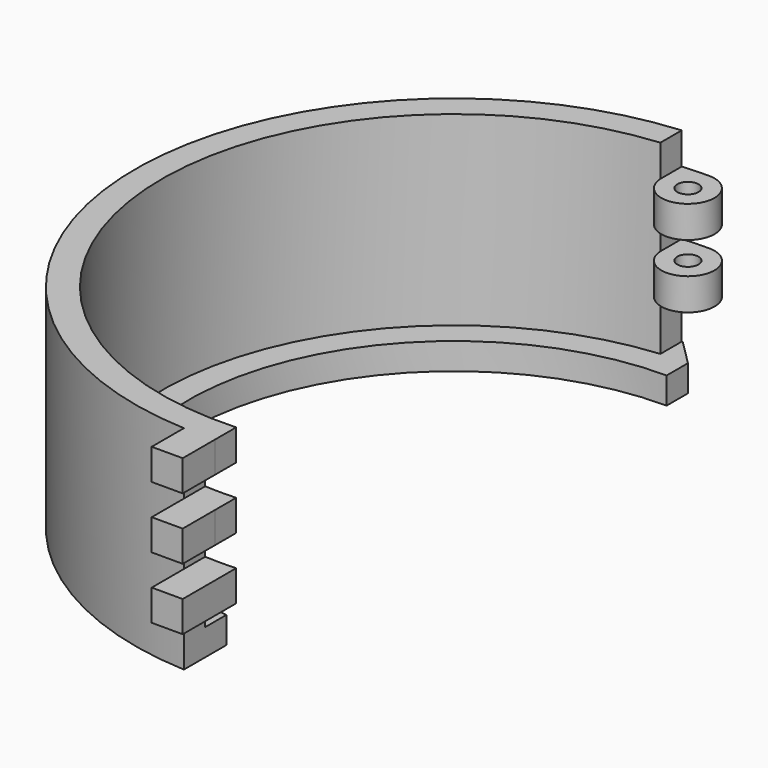
from build123d import *

# Parameters (mm, degrees)
F3_W           = 1.8520833333
F3_H           = 3.7041666667
F3_H_2         = 3.175
F4_DEPTH       = 38.1
F6_DEPTH       = 25.401
F7_R           = 3.175
F8_DEPTH       = 15.24
F9_R           = 1.27
F10_DEPTH      = 22.225
F11_W          = 3.175
F11_H          = 3.81
F11_H_2        = 6.985
F12_DEPTH      = 3.175
F13_DEPTH      = 4.7625
F13_DEPTH_BACK = 3.175
F15_DEPTH      = 3.175


# Not quite as in the source:
# - a length typed as a fraction of an inch, garbled in the dataset ("3 / 203.2 mm" for 3/8 in), is restored
# - a feature names something its author has since deleted; it is built from what else it names


with BuildPart() as f1:
    # F0 (on Front) → F1 (revolve)
    with BuildSketch(Plane.XZ):
        Polygon((-38.1, 0), (-31.75, 0), (-31.75, 3.175), (-34.925, 3.175), (-34.925, 25.4), (-38.1, 25.4), align=None)
    revolve(axis=Axis((0, 0, 12.7), (0, 0, 1)))

    # F3 (on offset) → F4 (cut, symmetric)
    with BuildSketch(Plane.XZ.offset(38.1)):
        with Locations((-0.9260416667, 5.0270833333)):
            Rectangle(F3_W, F3_H)
        with Locations((0.9260416667, 5.0270833333)):
            Rectangle(F3_W, F3_H)
        with Locations((0.9260416667, 12.4354166667)):
            Rectangle(F3_W, F3_H)
        with Locations((-0.9260416667, 12.4354166667)):
            Rectangle(F3_W, F3_H)
        with Locations((-0.9260416667, 19.84375)):
            Rectangle(F3_W, F3_H)
        Polygon((1.8520833333, 3.175), (1.8520833333, 0), (50.8, 0), (50.8, 25.4), (1.8520833333, 25.4), (1.8520833333, 21.6958333333), (1.8520833333, 17.9916666667), (1.8520833333, 14.2875), (1.8520833333, 10.5833333333), (1.8520833333, 6.8791666667), align=None)
        with Locations((0.9260416667, 19.84375)):
            Rectangle(F3_W, F3_H)
        with Locations((0.9260416667, 1.5875)):
            Rectangle(F3_W, F3_H_2)
        with Locations((-0.9260416667, 1.5875)):
            Rectangle(F3_W, F3_H_2)
    extrude(amount=F4_DEPTH, both=True, mode=Mode.SUBTRACT)

    # F5 (on face) → F6 (cut, through all)
    with BuildSketch(Plane.XY.offset(25.4)):
        with BuildLine():
            ThreePointArc((0, 38.1), (3.175, 34.925), (0, 31.75))
            ThreePointArc((0, 31.75), (22.4506403027, 22.4506403027), (31.75, 0))
            Line((31.75, 0), (41.275, 0))
            ThreePointArc((41.275, 0), (27.0107441469, 31.2096992237), (-5.922835282, 40.847835282))
            Line((-5.922835282, 40.847835282), (-3.0525211735, 37.9775211735))
            ThreePointArc((-3.0525211735, 37.9775211735), (-1.5274886724, 38.0693679795), (0, 38.1))
        make_face()
    extrude(amount=-F6_DEPTH, mode=Mode.SUBTRACT)

    # F7 (on face) → F8 (join)
    with BuildSketch(Plane.XY.offset(25.4)):
        with Locations((0, 34.925)):
            Circle(F7_R)
    extrude(amount=-F8_DEPTH)

    # F9 (on face) → F10 (cut)
    with BuildSketch(Plane.XY.offset(25.4)):
        with Locations((0, 34.925)):
            Circle(F9_R)
    extrude(amount=-F10_DEPTH, mode=Mode.SUBTRACT)

    # F11 (on Right) → F12 (cut, symmetric)
    with BuildSketch(Plane.YZ):
        with Locations((36.5125, 23.495)):
            Rectangle(F11_W, F11_H)
        with Locations((33.3375, 23.495)):
            Rectangle(F11_W, F11_H)
        with Locations((36.5125, 15.875)):
            Rectangle(F11_W, F11_H)
        with Locations((36.5125, 6.6675)):
            Rectangle(F11_W, F11_H_2)
        with Locations((33.3375, 6.6675)):
            Rectangle(F11_W, F11_H_2)
        with Locations((33.3375, 15.875)):
            Rectangle(F11_W, F11_H)
    extrude(amount=F12_DEPTH, both=True, mode=Mode.SUBTRACT)

    # F3 (on offset) → F13 (join, two sides)
    with BuildSketch(Plane.XZ.offset(38.1)) as f13_sk:
        with Locations((-0.9260416667, 8.73125)):
            Rectangle(F3_W, F3_H)
        with Locations((0.9260416667, 8.73125)):
            Rectangle(F3_W, F3_H)
        with Locations((-0.9260416667, 16.1395833333)):
            Rectangle(F3_W, F3_H)
        with Locations((0.9260416667, 16.1395833333)):
            Rectangle(F3_W, F3_H)
        with Locations((-0.9260416667, 23.5479166667)):
            Rectangle(F3_W, F3_H)
        with Locations((0.9260416667, 23.5479166667)):
            Rectangle(F3_W, F3_H)
    extrude(amount=F13_DEPTH)
    extrude(f13_sk.sketch, amount=-F13_DEPTH_BACK)

    # F14 (on face) → F15 (cut)
    with BuildSketch(Plane(origin=(0, 0, 0), x_dir=(1, 0, 0), z_dir=(0, 0, -1))):
        with BuildLine():
            Line((0, -31.75), (0, -34.925))
            Line((0, -34.925), (-3.0525211735, -37.9775211735))
            ThreePointArc((-3.0525211735, -37.9775211735), (-1.5274886724, -38.0693679795), (0, -38.1))
            ThreePointArc((0, -38.1), (3.175, -34.925), (0, -31.75))
        make_face()
    extrude(amount=-F15_DEPTH, mode=Mode.SUBTRACT)


solid = f1.part
